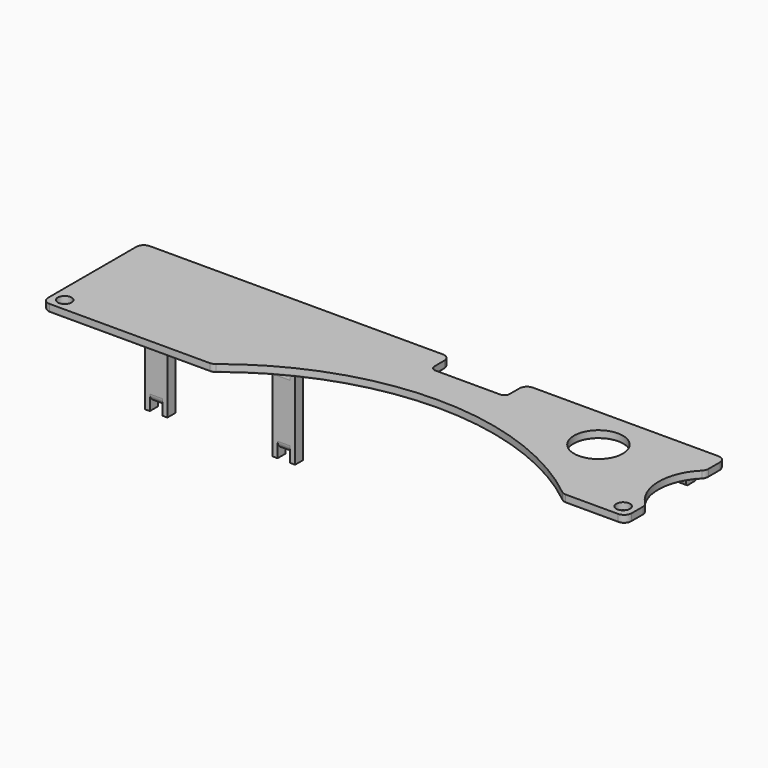
from build123d import *

# Parameters (mm, degrees)
F0_R      = 2.75
F0_R_2    = 9.75
F0_W      = 5
F0_H      = 4
F0_W_2    = 2
F0_H_2    = 1.3
F0_W_3    = 3
F0_H_3    = 3
F0_H_4    = 1.2
F1_DEPTH  = 3
F2_DEPTH  = 4
F3_START  = -4
F3_DEPTH  = 2
F4_DEPTH  = 35
F5_START  = -3
F5_DEPTH  = 29
F6_R      = 3
F7_R      = 0.5
F8_R      = 1
F9_DEPTH  = 4
F10_START = -4
F10_DEPTH = 2
F11_R     = 1


# Not quite as in the source:
# - a feature names something its author has since deleted; it is built from what else it names


with BuildPart() as f1:
    # F0 (on Top) → F1 (new body)
    with BuildSketch(Plane.XY):
        with BuildLine():
            Line((13, 40), (0, 40))
            Line((0, 40), (-13, 40))
            ThreePointArc((-13, 40), (-14.4142135624, 40.5857864376), (-15, 42))
            Line((-15, 42), (-15, 47))
            ThreePointArc((-15, 47), (-15.8786796564, 49.1213203436), (-18, 50))
            Line((-18, 50), (-128, 50))
            Line((-128, 50), (-135, 50))
            ThreePointArc((-135, 50), (-137.1213203436, 49.1213203436), (-138, 47))
            Line((-138, 47), (-138, 3))
            ThreePointArc((-138, 3), (-137.1213203436, 0.8786796564), (-135, 0))
            Line((-135, 0), (-128, 0))
            Line((-128, 0), (-71.0633520178, 0))
            ThreePointArc((-71.0633520178, 0), (-70.0677670504, 0.1700157999), (-69.1850255327, 0.6607929515))
            ThreePointArc((-69.1850255327, 0.6607929515), (0, 25), (69.1850255327, 0.6607929515))
            ThreePointArc((69.1850255327, 0.6607929515), (70.0677670504, 0.1700157999), (71.0633520178, 0))
            Line((71.0633520178, 0), (85, 0))
            Line((85, 0), (92, 0))
            ThreePointArc((92, 0), (94.1213203436, 0.8786796564), (95, 3))
            Line((95, 3), (95, 8.7019184973))
            ThreePointArc((95, 8.7019184973), (94.7704135973, 9.8529217554), (94.1167943333, 10.8277552151))
            ThreePointArc((94.1167943333, 10.8277552151), (88.2287565553, 25), (94.1167943333, 39.1722447849))
            ThreePointArc((94.1167943333, 39.1722447849), (94.7704135973, 40.1470782446), (95, 41.2980815027))
            Line((95, 41.2980815027), (95, 47))
            ThreePointArc((95, 47), (94.1213203436, 49.1213203436), (92, 50))
            Line((92, 50), (85, 50))
            Line((85, 50), (18, 50))
            ThreePointArc((18, 50), (15.8786796564, 49.1213203436), (15, 47))
            Line((15, 47), (15, 42))
            ThreePointArc((15, 42), (14.4142135624, 40.5857864376), (13, 40))
        make_face()
        with Locations((-133, 5)):
            Circle(F0_R, mode=Mode.SUBTRACT)
        Polygon((-111, 20), (-113, 20), (-113, 24), (-111, 24), (-106, 24), (-104, 24), (-104, 20), (-106, 20), align=None, mode=Mode.SUBTRACT)
        Polygon((-53, 24), (-53, 20), (-55, 20), (-60, 20), (-62, 20), (-62, 24), (-60, 24), (-55, 24), align=None, mode=Mode.SUBTRACT)
        with Locations((90, 5)):
            Circle(F0_R, mode=Mode.SUBTRACT)
        Polygon((-41.7887758017, 31), (-43.7887758017, 31), (-43.7887758017, 32.3), (-43.7887758017, 36.3), (-43.7887758017, 37.6), (-41.7887758017, 37.6), (-41.7887758017, 36.3), (-41.7887758017, 32.3), align=None, mode=Mode.SUBTRACT)
        Polygon((29, 31), (27, 31), (27, 32.3), (27, 36.3), (27, 37.6), (29, 37.6), (29, 36.3), (29, 32.3), align=None, mode=Mode.SUBTRACT)
        with Locations((57.9733885825, 32.6971039176)):
            Circle(F0_R_2, mode=Mode.SUBTRACT)
        Polygon((86, 42.4980815027), (86, 41.2980815027), (83, 41.2980815027), (83, 42.4980815027), (83, 45.4980815027), (83, 46.6980815027), (86, 46.6980815027), (86, 45.4980815027), align=None, mode=Mode.SUBTRACT)
        with Locations((-108.5, 22)):
            Rectangle(F0_W, F0_H)
        with Locations((-112, 22)):
            Rectangle(F0_W_2, F0_H)
        with Locations((-105, 22)):
            Rectangle(F0_W_2, F0_H)
        with Locations((-57.5, 22)):
            Rectangle(F0_W, F0_H)
        with Locations((-61, 22)):
            Rectangle(F0_W_2, F0_H)
        with Locations((-54, 22)):
            Rectangle(F0_W_2, F0_H)
        with Locations((-42.7887758017, 34.3)):
            Rectangle(F0_W_2, F0_H)
        with Locations((-42.7887758017, 31.65)):
            Rectangle(F0_W_2, F0_H_2)
        with Locations((-42.7887758017, 36.95)):
            Rectangle(F0_W_2, F0_H_2)
        with Locations((28, 34.3)):
            Rectangle(F0_W_2, F0_H)
        with Locations((28, 31.65)):
            Rectangle(F0_W_2, F0_H_2)
        with Locations((28, 36.95)):
            Rectangle(F0_W_2, F0_H_2)
        with Locations((84.5, 43.9980815027)):
            Rectangle(F0_W_3, F0_H_3)
        with Locations((84.5, 46.0980815027)):
            Rectangle(F0_W_3, F0_H_4)
        with Locations((84.5, 41.8980815027)):
            Rectangle(F0_W_3, F0_H_4)
    extrude(amount=F1_DEPTH)

    # F0 (on Top) → F2 (join)
    with BuildSketch(Plane.XY):
        with Locations((-42.7887758017, 36.95)):
            Rectangle(F0_W_2, F0_H_2)
        with Locations((-42.7887758017, 31.65)):
            Rectangle(F0_W_2, F0_H_2)
        with Locations((28, 31.65)):
            Rectangle(F0_W_2, F0_H_2)
        with Locations((28, 36.95)):
            Rectangle(F0_W_2, F0_H_2)
    extrude(amount=-F2_DEPTH)

    # F0 (on Top) → F3 (join)
    with BuildSketch(Plane.XY.offset(F3_START)):
        with Locations((-42.7887758017, 34.3)):
            Rectangle(F0_W_2, F0_H)
        with Locations((-42.7887758017, 36.95)):
            Rectangle(F0_W_2, F0_H_2)
        with Locations((-42.7887758017, 31.65)):
            Rectangle(F0_W_2, F0_H_2)
        with Locations((28, 34.3)):
            Rectangle(F0_W_2, F0_H)
        with Locations((28, 36.95)):
            Rectangle(F0_W_2, F0_H_2)
        with Locations((28, 31.65)):
            Rectangle(F0_W_2, F0_H_2)
    extrude(amount=-F3_DEPTH)

    # F0 (on Top) → F4 (join)
    with BuildSketch(Plane.XY):
        with Locations((-112, 22)):
            Rectangle(F0_W_2, F0_H)
        with Locations((-105, 22)):
            Rectangle(F0_W_2, F0_H)
        with Locations((-61, 22)):
            Rectangle(F0_W_2, F0_H)
        with Locations((-54, 22)):
            Rectangle(F0_W_2, F0_H)
    extrude(amount=-F4_DEPTH)

    # F0 (on Top) → F5 (join)
    with BuildSketch(Plane.XY.offset(F5_START)):
        with Locations((-108.5, 22)):
            Rectangle(F0_W, F0_H)
        with Locations((-57.5, 22)):
            Rectangle(F0_W, F0_H)
    extrude(amount=-F5_DEPTH)

    # F6
    f6_edges = [f1.edges().sort_by_distance(p)[0] for p in [
        (-57.5, 20, -32),
        (-57.5, 20, -3),
        (-108.5, 20, -32),
        (-108.5, 20, -3),
    ]]
    fillet(f6_edges, radius=F6_R)

    # F7
    f7_edges = [f1.edges().sort_by_distance(p)[0] for p in [
        (-103.031676, 0, 0),
        (-135.75, 5, 0),
        (48.223389, 32.697104, 0),
        (87.25, 5, 0),
        (-57.5, 24, -32),
        (-57.5, 24, -3),
        (-108.5, 24, -3),
        (-108.5, 24, -32),
    ]]
    fillet(f7_edges, radius=F7_R)

    # F8
    f8_edges = [f1.edges().sort_by_distance(p)[0] for p in [
        (-42.788776, 32.3, 0),
        (-42.788776, 36.3, 0),
        (28, 32.3, 0),
        (-42.788776, 36.3, -4),
        (-42.788776, 32.3, -4),
        (28, 32.3, -4),
        (28, 36.3, 0),
        (28, 36.3, -4),
        (28, 31, -6),
        (28, 37.6, -6),
        (28, 37.6, 0),
        (28, 31, 0),
        (-42.788776, 37.6, -6),
        (-42.788776, 37.6, 0),
        (-42.788776, 31, 0),
        (-42.788776, 31, -6),
        (-62, 22, 0),
        (-53, 22, 0),
        (-113, 22, 0),
        (-104, 22, 0),
    ]]
    fillet(f8_edges, radius=F8_R)

    # F0 (on Top) → F9 (join)
    with BuildSketch(Plane.XY):
        with Locations((84.5, 41.8980815027)):
            Rectangle(F0_W_3, F0_H_4)
        with Locations((84.5, 46.0980815027)):
            Rectangle(F0_W_3, F0_H_4)
    extrude(amount=-F9_DEPTH)

    # F0 (on Top) → F10 (join)
    with BuildSketch(Plane.XY.offset(F10_START)):
        with Locations((84.5, 43.9980815027)):
            Rectangle(F0_W_3, F0_H_3)
        with Locations((84.5, 41.8980815027)):
            Rectangle(F0_W_3, F0_H_4)
        with Locations((84.5, 46.0980815027)):
            Rectangle(F0_W_3, F0_H_4)
    extrude(amount=-F10_DEPTH)

    # F11
    f11_edges = [f1.edges().sort_by_distance(p)[0] for p in [
        (84.5, 41.298082, -6),
        (84.5, 46.698082, -6),
        (84.5, 42.498082, -4),
        (84.5, 45.498082, -4),
        (84.5, 45.498082, 0),
        (84.5, 42.498082, 0),
        (84.5, 41.298082, 0),
        (84.5, 46.698082, 0),
    ]]
    fillet(f11_edges, radius=F11_R)


solid = f1.part
